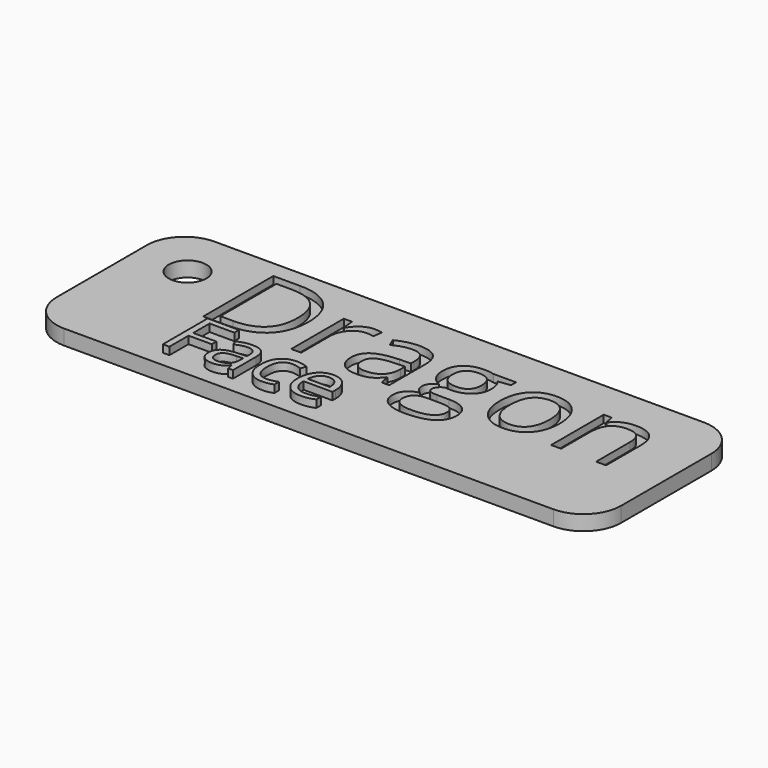
from build123d import *

# Parameters (mm, degrees)
F1_DEPTH     = 2
F3_D         = 5
F4_TEXT_SIZE = 16.3181815852
F5_DEPTH     = 1
F6_TEXT_SIZE = 10.4201456306
F7_DEPTH     = 1


# Not quite as in the source:
# - Text() gives the source's letters only with a copy of the font that has no kerning and outlines rounded to 1/6400 em; it was checked with that copy


with BuildPart() as f1:
    # F0 (on Top) → F1 (new body)
    with BuildSketch(Plane.XY):
        with BuildLine():
            Line((32.5, 12.5), (-32.5, 12.5))
            ThreePointArc((-32.5, 12.5), (-36.0355339059, 11.0355339059), (-37.5, 7.5))
            Line((-37.5, 7.5), (-37.5, -7.5))
            ThreePointArc((-37.5, -7.5), (-36.0355339059, -11.0355339059), (-32.5, -12.5))
            Line((-32.5, -12.5), (32.5, -12.5))
            ThreePointArc((32.5, -12.5), (36.0355339059, -11.0355339059), (37.5, -7.5))
            Line((37.5, -7.5), (37.5, 7.5))
            ThreePointArc((37.5, 7.5), (36.0355339059, 11.0355339059), (32.5, 12.5))
        make_face()
    extrude(amount=F1_DEPTH)

    # F3 (through all)
    with Locations(Plane.XY.offset(2)):
        with Locations((-30.5, 5.5)):
            Hole(F3_D / 2)

    # F4 (on face) → F5 (cut)
    with BuildSketch(Plane.XY.offset(2)):
        with Locations((-24.5257607102, -1.3760700115)):
            Text('Dragon', F4_TEXT_SIZE, font='Open Sans', text_align=(TextAlign.LEFT, TextAlign.BOTTOM))
    extrude(amount=-F5_DEPTH, mode=Mode.SUBTRACT)

    # F6 (on face) → F7 (join)
    with BuildSketch(Plane.XY.offset(2)):
        with Locations((-22.1102465099, -10.3599597876)):
            Text('Face', F6_TEXT_SIZE, font='Open Sans', text_align=(TextAlign.LEFT, TextAlign.BOTTOM))
    extrude(amount=F7_DEPTH)


solid = f1.part
